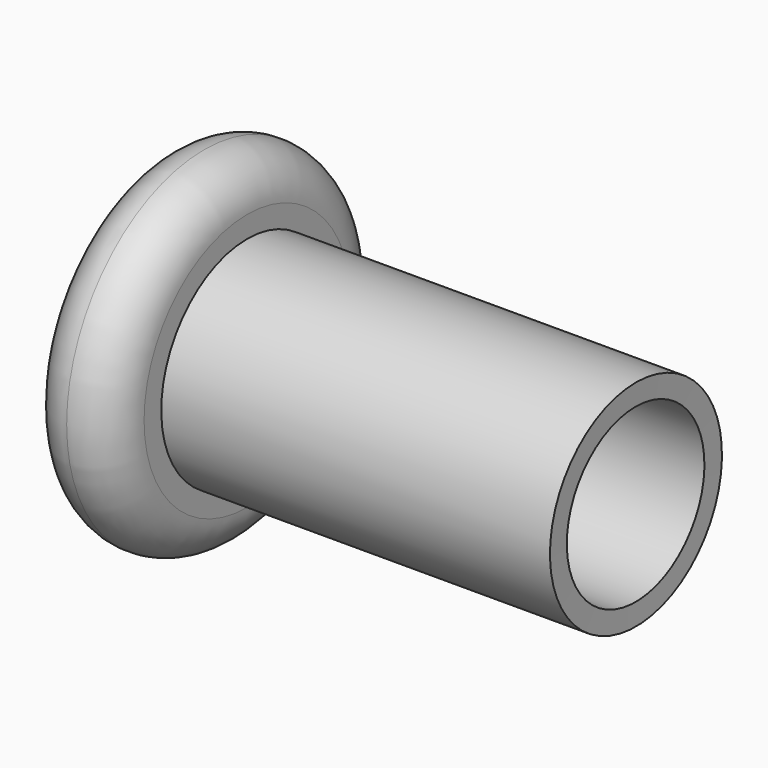
from build123d import *

# Parameters (mm, degrees)
F4_R = 0.99999
F3_T = -0.5


# Not quite as in the source:
# - a fillet or chamfer is up to 0.001 mm smaller than in the source, because OpenCascade refuses the exact size


with BuildPart() as f2:
    # F0 (on Front) → F2 (revolve)
    with BuildSketch(Plane.XZ):
        Polygon((0, 4), (0, 0), (11, 0), (11.0396612436, 2.5), (2, 2.5), (2, 4), align=None)
    revolve(axis=Axis((6.7295320332, 0, 0), (1, 0, 0)))

    # F4 (radius 1 in the source; OpenCascade refuses exactly that, so slightly less here)
    f4_edges = [f2.edges().sort_by_distance(p)[0] for p in [
        (2, 0, -4),
        (0, 0, -4),
    ]]
    fillet(f4_edges, radius=F4_R)

    # F3
    f3_openings = [f2.faces().sort_by_distance(p)[0] for p in [
        (11.019831, 0, -1.25),
    ]]
    offset(amount=F3_T, openings=f3_openings, kind=Kind.INTERSECTION)


solid = f2.part
